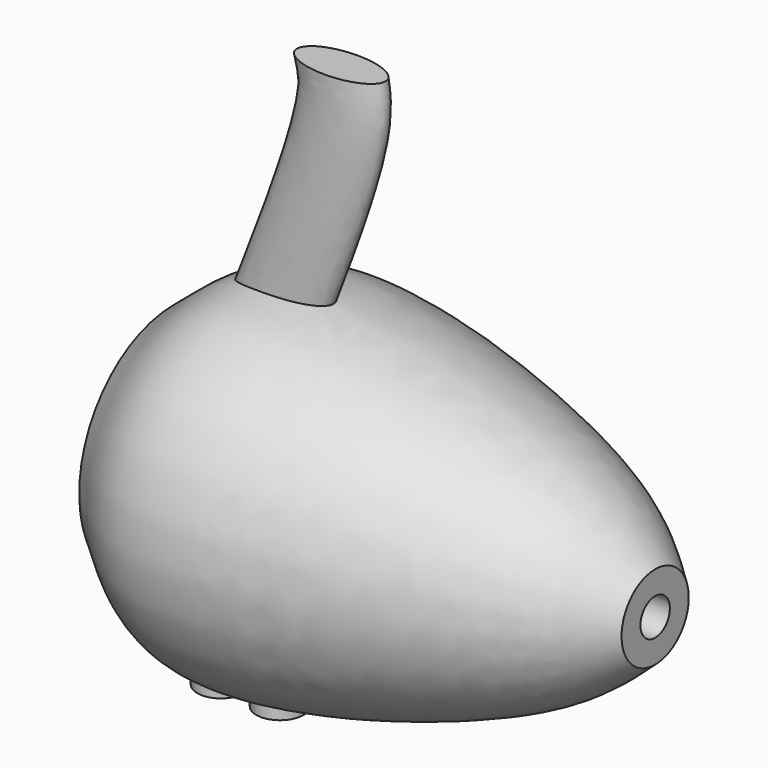
from build123d import *

# Parameters (mm, degrees)
F3_R     = 10.16
F4_DEPTH = 35.56


# Not quite as in the source:
# - a feature names something its author has since deleted; it is built from what else it names


with BuildPart() as f1:
    # F0 (on Front) → F1 (revolve)
    with BuildSketch(Plane.XZ):
        with BuildLine():
            Line((207.1336402178, -42.8901373174), (207.1336402178, -32.7301373174))
            add(Edge.make_bspline(
                [(0, 0), (10.4638618624, 8.1276784662), (33.2666475246, 37.2417350062), (163.1452860385, 2.6466282002), (191.1877777142, -17.7927619281), (207.1336402178, -32.7301373174)],
                knots=[0, 0, 0, 0, 0.2590203832, 0.6935859965, 1, 1, 1, 1], degree=3))
            Line((0, 0), (0, -25.4))
            Line((0, -25.4), (76.2, -25.4))
            Line((76.2, -25.4), (76.2, -15.24))
            Line((76.2, -15.24), (152.4, -15.24))
            Line((152.4, -15.24), (181.8301071367, -32.7301373174))
            Line((181.8301071367, -32.7301373174), (181.8301071367, -42.8901373174))
            Line((181.8301071367, -42.8901373174), (207.1336402178, -42.8901373174))
        make_face()
    revolve(axis=Axis((71.7367434391, 0, -50.8), (-1, 0, 0)))

    # F3 (on offset) → F4 (join)
    with BuildSketch(Plane.XY.offset(-101.6)):
        with Locations((20.32, 0)):
            Circle(F3_R)
        with Locations((45.72, 0)):
            Circle(F3_R)
    extrude(amount=-F4_DEPTH)

    # F8: sweep along a path in F5
    with BuildLine(Plane.XZ) as f8_path:
        add(Plane.XZ * Edge.make_bspline(
            [(39.8880077945, 0), (54.9183498543, 38.4224136512), (76.2580250899, 92.973522723), (73.0281734091, 109.4334294306), (72.0732286811, 114.3)],
            knots=[0, 0, 0, 0, 0.7043379008, 1, 1, 1, 1], degree=3))
    # F7 (on offset) → F8 (sweep)
    with BuildSketch(Plane.XY.offset(114.3)):
        with BuildLine():
            add(Edge.make_bspline(
                [(53.0232286811, 0), (53.0232286811, -15.3979316793), (81.5982286811, -7.6989658396), (110.1732286811, 0), (81.5982286811, 7.6989658396), (53.0232286811, 15.3979316793), (53.0232286811, 0)],
                knots=[0, 0, 0, 2.0943951024, 2.0943951024, 4.1887902048, 4.1887902048, 6.2831853072, 6.2831853072, 6.2831853072], degree=2, weights=[1, 0.5, 1, 0.5, 1, 0.5, 1]))
        make_face()
    sweep(path=f8_path.line)


solid = f1.part
